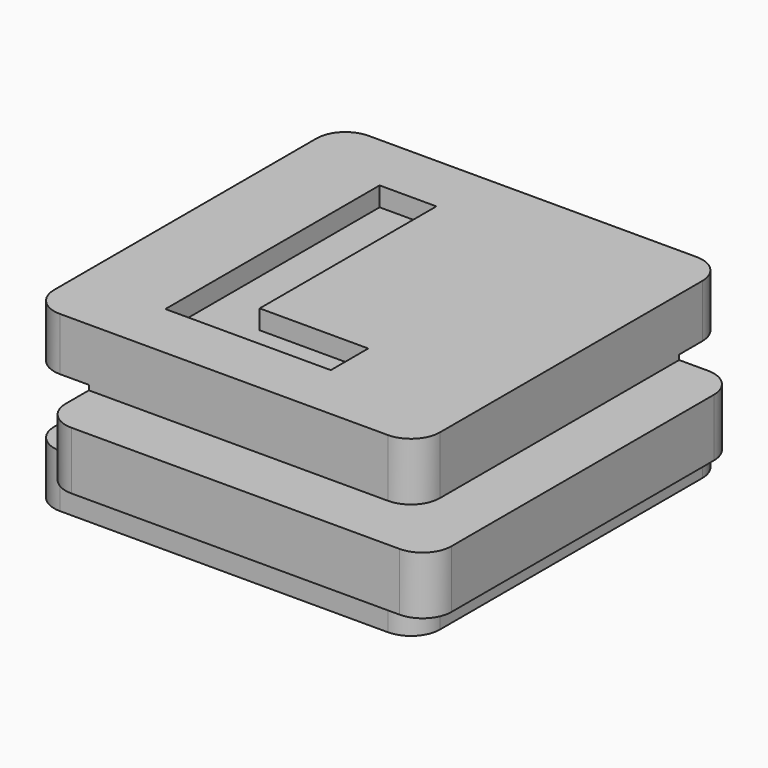
from build123d import *

# Parameters (mm, degrees)
F0_W         = 14
F0_H         = 3
F0_W_2       = 3
F1_DEPTH     = 20
F2_DEPTH     = 3
F3_W         = 3
F3_H         = 3
F4_DEPTH     = 100
F5_W         = 3
F5_H         = 3.5
F6_DEPTH     = 100
F7_R         = 1.5
F8_TEXT_SIZE = 19.4444444444
F9_DEPTH     = 1


# Not quite as in the source:
# - Text() gives the source's letters only with a copy of the font that has no kerning and outlines rounded to 1/6400 em; it was checked with that copy


with BuildPart() as f1:
    # F0 (on Front) → F1 (new body)
    with BuildSketch(Plane.XZ):
        Polygon((10, 1.5), (10, 4.5), (-10, 4.5), (-10, 1.5), (-7, 1.5), (7, 1.5), align=None)
        Rectangle(F0_W, F0_H)
        with Locations((11.5, 0)):
            Rectangle(F0_W_2, F0_H)
        with Locations((8.5, 0)):
            Rectangle(F0_W_2, F0_H)
        with Locations((-8.5, 0)):
            Rectangle(F0_W_2, F0_H)
        Polygon((10, -4.5), (10, -1.5), (7, -1.5), (-7, -1.5), (-10, -1.5), (-10, -4.5), align=None)
    extrude(amount=-F1_DEPTH)

    # F0 (on Front) → F2 (join)
    with BuildSketch(Plane.XZ):
        with Locations((-8.5, 0)):
            Rectangle(F0_W_2, F0_H)
        Rectangle(F0_W, F0_H)
        with Locations((8.5, 0)):
            Rectangle(F0_W_2, F0_H)
        with Locations((11.5, 0)):
            Rectangle(F0_W_2, F0_H)
    extrude(amount=F2_DEPTH)

    # F3 (on face) → F4 (cut)
    with BuildSketch(Plane.YZ.offset(13)):
        Polygon((23, -1.75), (23, 1.75), (17, 1.75), (17, 1.5), (20, 1.5), (20, -1.5), (17, -1.5), (17, -1.75), align=None)
        with Locations((18.5, 0)):
            Rectangle(F3_W, F3_H)
    extrude(amount=-F4_DEPTH, mode=Mode.SUBTRACT)

    # F5 (on face) → F6 (cut)
    with BuildSketch(Plane(origin=(0, 17, 0), x_dir=(-1, 0, 0), z_dir=(0, 1, 0))):
        with Locations((11.5, 0)):
            Rectangle(F5_W, F5_H)
        with Locations((8.5, 0)):
            Rectangle(F5_W, F5_H)
    extrude(amount=-F6_DEPTH, mode=Mode.SUBTRACT)

    # F7
    f7_edges = [f1.edges().sort_by_distance(p)[0] for p in [
        (-7, -3, 0),
        (13, -3, 0),
        (10, 0, 3),
        (10, 0, -3),
        (-10, 0, -3.125),
        (-10, 0, 3.125),
        (-7, 17, 0),
        (-10, 20, 3.125),
        (-10, 20, -3.125),
        (13, 17, 0),
        (10, 20, 3.125),
        (10, 20, -3.125),
    ]]
    fillet(f7_edges, radius=F7_R)

    # F8 (on face) → F9 (cut)
    with BuildSketch(Plane.XY.offset(4.5)):
        with Locations((-7.1801951318, 3)):
            Text('L', F8_TEXT_SIZE, font='Open Sans', font_style=FontStyle.BOLD, text_align=(TextAlign.LEFT, TextAlign.BOTTOM))
    extrude(amount=-F9_DEPTH, mode=Mode.SUBTRACT)


solid = f1.part
